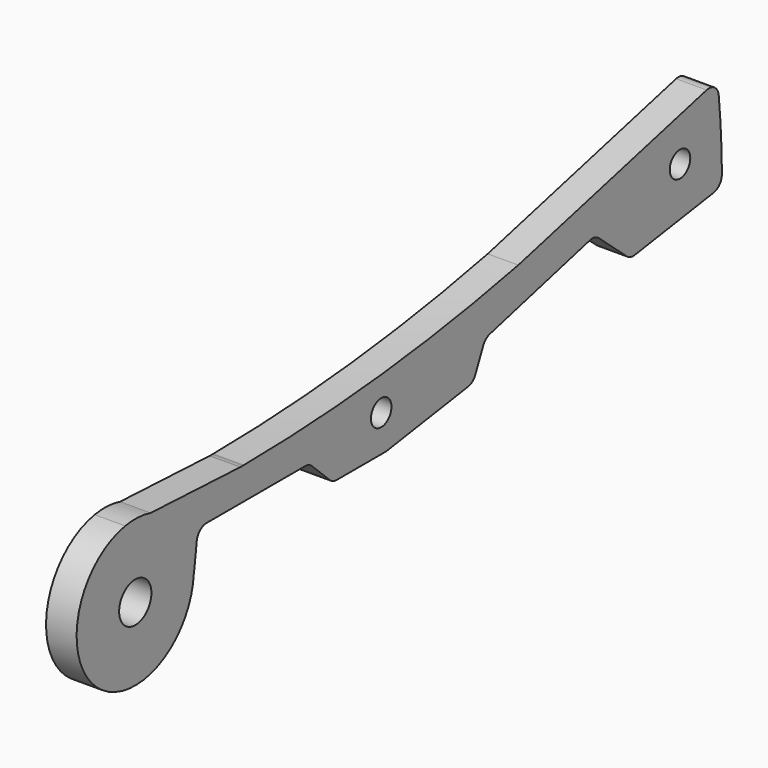
from build123d import *

# Parameters (mm, degrees)
F0_R     = 3.3
F0_R_2   = 2.1
F1_DEPTH = 5


# Not quite as in the source:
# - a feature names something its author has since deleted; it is built from what else it names


with BuildPart() as f1:
    # F0 (on Right) → F1 (new body)
    with BuildSketch(Plane.YZ):
        with BuildLine():
            ThreePointArc((21.8315579223, 10.717182122), (21.897134346, 10.7177196915), (21.9626931438, 10.7193322557))
            ThreePointArc((21.9626931438, 10.7193322557), (21.9630378123, 10.7252568669), (21.9633808826, 10.731181571))
            ThreePointArc((21.9633808826, 10.731181571), (21.7716697335, 10.7299327404), (21.5799577929, 10.728811993))
            Line((21.5799577929, 10.728811993), (21.8315579223, 10.717182122))
        make_face()
        with BuildLine():
            ThreePointArc((22.1844688263, 10.7327808001), (22.0736743793, 10.7245163933), (21.9626931438, 10.7193322557))
            ThreePointArc((21.9626931438, 10.7193322557), (21.897134346, 10.7177196915), (21.8315579223, 10.717182122))
            ThreePointArc((21.8315579223, 10.717182122), (21.6468606164, 10.7214485341), (21.4625573078, 10.7342386694))
            Line((21.4625573078, 10.7342386694), (3.1432257368, 11.581024651))
            Line((3.1432257368, 11.581024651), (-2.0614712889, 11.8216046341))
            ThreePointArc((-2.0614712889, 11.8216046341), (-7.9885695505, -8.9544824829), (11.9792964571, -0.7045966171))
            ThreePointArc((11.9792964571, -0.7045966171), (12.0074816864, -0.4822378377), (12.0652655082, -0.2656763826))
            Line((12.0652655082, -0.2656763826), (12.5823545671, 3.7402298466))
            ThreePointArc((12.5823545671, 3.7402298466), (13.2453067327, 4.9862024463), (14.565897859, 5.4841907695))
            Line((14.565897859, 5.4841907695), (34.746018001, 5.4841907695))
            ThreePointArc((34.746018001, 5.4841907695), (35.4911723527, 5.3401931919), (36.1290262829, 4.9289357615))
            Line((36.1290262829, 4.9289357615), (39.7961525429, 1.4185128035))
            ThreePointArc((39.7961525429, 1.4185128035), (40.4340064731, 1.0072553731), (41.1791608249, 0.8632577956))
            Line((41.1791608249, 0.8632577956), (51.1560065331, 0.8632577956))
            ThreePointArc((51.1560065331, 0.8632577956), (51.3046360431, 0.8687881245), (51.452443583, 0.8853485268))
            Line((51.452443583, 0.8853485268), (68.043755982, 3.3719538424))
            ThreePointArc((68.043755982, 3.3719538424), (68.9480745213, 3.750430082), (69.5639006382, 4.5131846154))
            Line((69.5639006382, 4.5131846154), (71.1927053136, 8.0496168184))
            ThreePointArc((71.1927053136, 8.0496168184), (71.7304115705, 8.7506241115), (72.5176709464, 9.151575379))
            Line((72.5176709464, 9.151575379), (93.0016589096, 14.3460792675))
            ThreePointArc((93.0016589096, 14.3460792675), (93.9531599103, 14.3538506609), (94.800564285, 13.9210454222))
            Line((94.800564285, 13.9210454222), (100.5567479715, 8.9494668086))
            ThreePointArc((100.5567479715, 8.9494668086), (101.3078443235, 8.5419637232), (102.1604743235, 8.4851607509))
            Line((102.1604743235, 8.4851607509), (118.2931486533, 10.9030281733))
            ThreePointArc((118.2931486533, 10.9030281733), (119.516973098, 11.5813971433), (119.9966558679, 12.8958685851))
            ThreePointArc((119.9966558679, 12.8958685851), (119.8113324935, 18.7264110882), (119.3428752162, 24.5410579746))
            ThreePointArc((119.3428752162, 24.5410579746), (118.5020303548, 25.9696085801), (116.872434029, 26.2732411356))
            Line((116.872434029, 26.2732411356), (78.344444671, 16.7187866332))
            ThreePointArc((78.344444671, 16.7187866332), (50.4120849121, 12.3407543123), (22.1844688263, 10.7327808001))
        make_face()
        Circle(F0_R, mode=Mode.SUBTRACT)
        with Locations((50.3031872213, 6.8563437089)):
            Circle(F0_R_2, mode=Mode.SUBTRACT)
        with Locations((111.4225909114, 17.8264938295)):
            Circle(F0_R_2, mode=Mode.SUBTRACT)
        with BuildLine():
            ThreePointArc((21.9633808826, 10.731181571), (21.9630378123, 10.7252568669), (21.9626931438, 10.7193322557))
            ThreePointArc((21.9626931438, 10.7193322557), (22.0736743793, 10.7245163933), (22.1844688263, 10.7327808001))
            ThreePointArc((22.1844688263, 10.7327808001), (22.0739250085, 10.7319598925), (21.9633808826, 10.731181571))
        make_face()
        with BuildLine():
            ThreePointArc((21.4625573078, 10.7342386694), (21.6468606164, 10.7214485341), (21.8315579223, 10.717182122))
            Line((21.8315579223, 10.717182122), (21.5799577929, 10.728811993))
            Line((21.5799577929, 10.728811993), (21.4625573078, 10.7342386694))
        make_face()
        with BuildLine():
            Line((-2.0614712889, 11.8216046341), (3.1432257368, 11.581024651))
            ThreePointArc((3.1432257368, 11.581024651), (0.5540919179, 11.9872007636), (-2.0614712889, 11.8216046341))
        make_face()
    extrude(amount=F1_DEPTH)


solid = f1.part
